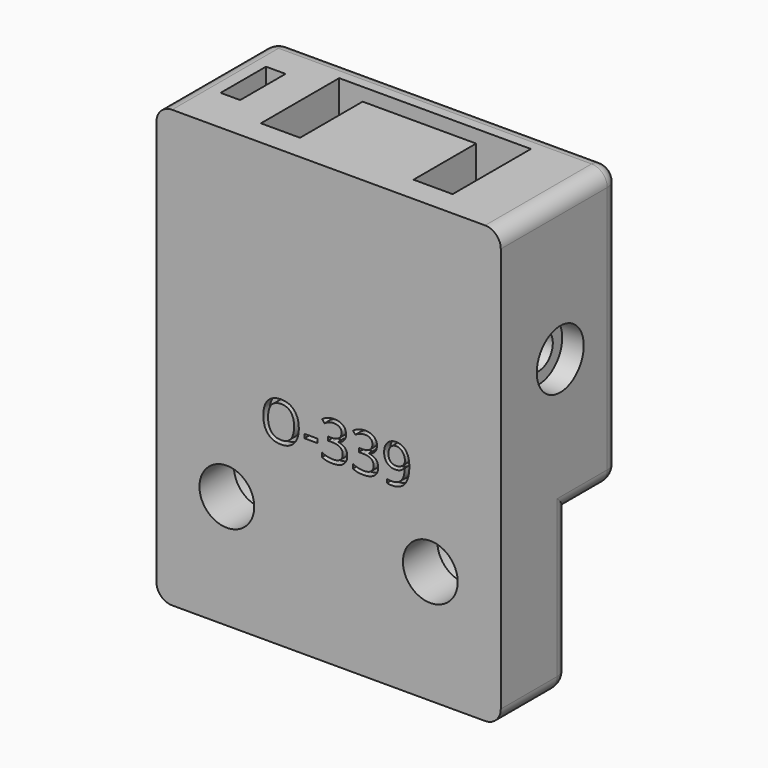
from build123d import *

# Parameters (mm, degrees)
F0_W          = 58
F0_H          = 19
F1_DEPTH      = 11
F2_W          = 58
F2_H          = 19
F3_DEPTH      = 24.75
F4_W          = 5
F4_H          = 12.5
F5_DEPTH      = 24.75
F6_R          = 2.25
F7_DEPTH      = 58.001
F8_W          = 14.5
F8_H          = 2.5
F9_DEPTH      = 24.75
F10_R         = 3.75
F11_DEPTH     = 10.75
F12_W         = 2.5
F12_H         = 7.25
F13_DEPTH     = 22
F14_TEXT_SIZE = 6.9078950522
F15_DEPTH     = 1
F16_W         = 58
F16_H         = 20
F17_DEPTH     = 11
F18_R         = 3.5
F19_DEPTH     = 11.0010001
F20_R         = 5.5
F21_DEPTH     = 5.5
F22_W         = 8
F22_H         = 55.75
F22_W_2       = 6
F23_DEPTH     = 19.0010001
F24_R         = 2


# Not quite as in the source:
# - Text() gives the source's letters only with a copy of the font that has no kerning and outlines rounded to 1/6400 em; it was checked with that copy


with BuildPart() as f1:
    # F0 (on Top) → F1 (new body)
    with BuildSketch(Plane.XY):
        Rectangle(F0_W, F0_H)
    extrude(amount=F1_DEPTH)

    # F2 (on face) → F3 (join)
    with BuildSketch(Plane.XY.offset(11)):
        Rectangle(F2_W, F2_H)
    extrude(amount=F3_DEPTH)

    # F4 (on face) → F5 (cut)
    with BuildSketch(Plane.XY.offset(35.75)):
        with Locations((-9.75, 0)):
            Rectangle(F4_W, F4_H)
        with Locations((9.75, 0)):
            Rectangle(F4_W, F4_H)
    extrude(amount=-F5_DEPTH, mode=Mode.SUBTRACT)

    # F6 (on face) → F7 (cut, through all)
    with BuildSketch(Plane.YZ.offset(29)):
        with Locations((0, 17.5)):
            Circle(F6_R)
    extrude(amount=-F7_DEPTH, mode=Mode.SUBTRACT)

    # F8 (on face) → F9 (cut)
    with BuildSketch(Plane.XY.offset(35.75)):
        with Locations((0, 5)):
            Rectangle(F8_W, F8_H)
    extrude(amount=-F9_DEPTH, mode=Mode.SUBTRACT)

    # F10 (on face) → F11 (cut)
    with BuildSketch(Plane.YZ.offset(29)):
        with Locations((0, 17.5)):
            Circle(F10_R)
    extrude(amount=-F11_DEPTH, mode=Mode.SUBTRACT)

    # F12 (on face) → F13 (cut)
    with BuildSketch(Plane.XY.offset(35.75)):
        with Locations((-18.25, 0)):
            Rectangle(F12_W, F12_H)
    extrude(amount=-F13_DEPTH, mode=Mode.SUBTRACT)

    # F14 (on face) → F15 (cut)
    with BuildSketch(Plane.XZ.offset(9.5)):
        with Locations((-9.7638779128, 2.6940791868)):
            Text('O-339', F14_TEXT_SIZE, font='Open Sans', text_align=(TextAlign.LEFT, TextAlign.BOTTOM))
    extrude(amount=-F15_DEPTH, mode=Mode.SUBTRACT)

    # F16 (on face) → F17 (join)
    with BuildSketch(Plane.XZ.offset(9.5)):
        with Locations((0, -10)):
            Rectangle(F16_W, F16_H)
    extrude(amount=-F17_DEPTH)

    # F18 (on face) → F19 (cut, through all)
    with BuildSketch(Plane(origin=(0, 1.5, 0), x_dir=(-1, 0, 0), z_dir=(0, 1, 0))):
        with Locations((-12, -5.5)):
            Circle(F18_R)
        with Locations((14, -5.5)):
            Circle(F18_R)
    extrude(amount=-F19_DEPTH, mode=Mode.SUBTRACT)

    # F20 (on face) → F21 (cut)
    with BuildSketch(Plane(origin=(0, 1.5, 0), x_dir=(-1, 0, 0), z_dir=(0, 1, 0))):
        with Locations((-12, -5.5)):
            Circle(F20_R)
        with Locations((14, -5.5)):
            Circle(F20_R)
    extrude(amount=-F21_DEPTH, mode=Mode.SUBTRACT)

    # F22 (on face) → F23 (cut, through all)
    with BuildSketch(Plane(origin=(0, 9.5, 0), x_dir=(-1, 0, 0), z_dir=(0, 1, 0))):
        with Locations((-25, 7.875)):
            Rectangle(F22_W, F22_H)
        with Locations((26, 7.875)):
            Rectangle(F22_W_2, F22_H)
    extrude(amount=-F23_DEPTH, mode=Mode.SUBTRACT)

    # F24
    f24_edges = [f1.edges().sort_by_distance(p)[0] for p in [
        (21, 1.5, -10),
        (-1, 1.5, -20),
        (21, -4, -20),
        (21, 5.5, 0),
        (21, 9.5, 17.875),
        (-1, 9.5, 0),
        (-23, 1.5, -10),
        (-23, -4, -20),
        (-23, 5.5, 0),
        (-23, 9.5, 17.875),
        (-1, 9.5, 35.75),
        (21, 0, 35.75),
        (-23, 0, 35.75),
    ]]
    fillet(f24_edges, radius=F24_R)


solid = f1.part
